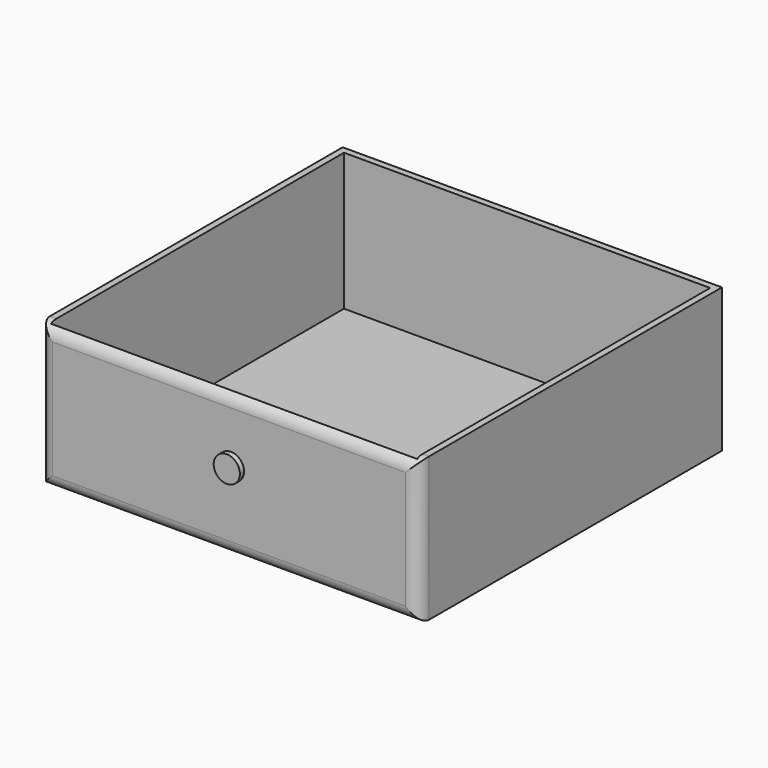
from build123d import *

# Parameters (mm, degrees)
F0_W        = 145
F0_H        = 145
F1_DEPTH    = 55
F2_T        = -2.5
F3_T1_DEPTH = 80
F3_T3_DEPTH = 170
F5_DEPTH    = 2


# Not quite as in the source:
# - a fillet or chamfer that OpenCascade refuses, or shapes differently, is made with other operations: its cross-section is extruded or revolved along the edge and cut away or added


with BuildPart() as f1:
    # F0 (on Top) → F1 (new body)
    with BuildSketch(Plane.XY):
        with Locations((-0.7837880796, -0.1337006688)):
            Rectangle(F0_W, F0_H)
    extrude(amount=F1_DEPTH)

    # F2
    f2_openings = [f1.faces().sort_by_distance(p)[0] for p in [
        (-0.783788, -0.133701, 55),
    ]]
    offset(amount=F2_T, openings=f2_openings)

    # F3: fillet of radius 5 on 4 edges, made by hand

    # F3_s2 → F3_t1 (cut)
    with BuildSketch(Plane.XY.offset(-12.5)):
        with BuildLine():
            ThreePointArc((-73.2837880796, -67.6337006688), (-71.8193219856, -71.1692345747), (-68.2837880796, -72.6337006688))
            Line((-68.2837880796, -72.6337006688), (-73.2837880796, -72.6337006688))
            Line((-73.2837880796, -72.6337006688), (-73.2837880796, -67.6337006688))
        make_face()
        with BuildLine():
            ThreePointArc((66.7162119204, -72.6337006688), (70.2517458263, -71.1692345747), (71.7162119204, -67.6337006688))
            Line((71.7162119204, -67.6337006688), (71.7162119204, -72.6337006688))
            Line((71.7162119204, -72.6337006688), (66.7162119204, -72.6337006688))
        make_face()
    extrude(amount=F3_T1_DEPTH, mode=Mode.SUBTRACT)

    # F3_s4 → F3_t3 (cut)
    with BuildSketch(Plane.YZ.offset(-85.7837880796)):
        with BuildLine():
            ThreePointArc((-72.6337006688, 5), (-71.1692345747, 1.4644660941), (-67.6337006688, 0))
            Line((-67.6337006688, 0), (-72.6337006688, 0))
            Line((-72.6337006688, 0), (-72.6337006688, 5))
        make_face()
        with BuildLine():
            ThreePointArc((-72.6337006688, 50), (-71.1692345747, 53.5355339059), (-67.6337006688, 55))
            Line((-67.6337006688, 55), (-72.6337006688, 55))
            Line((-72.6337006688, 55), (-72.6337006688, 50))
        make_face()
    extrude(amount=F3_T3_DEPTH, mode=Mode.SUBTRACT)

    # F4 (on face) → F5 (join)
    with BuildSketch(Plane.XZ.offset(72.6337006688)):
        with BuildLine():
            ThreePointArc((0, 25.2702692018), (3.5355339059, 26.7347352958), (5, 30.2702692018))
            ThreePointArc((5, 30.2702692018), (3.5355339059, 33.8058031077), (0, 35.2702692018))
            Line((0, 35.2702692018), (0, 25.2702692018))
        make_face()
        with BuildLine():
            Line((0, 25.2702692018), (0, 35.2702692018))
            ThreePointArc((0, 35.2702692018), (-5, 30.2702692018), (0, 25.2702692018))
        make_face()
    extrude(amount=F5_DEPTH)


solid = f1.part
